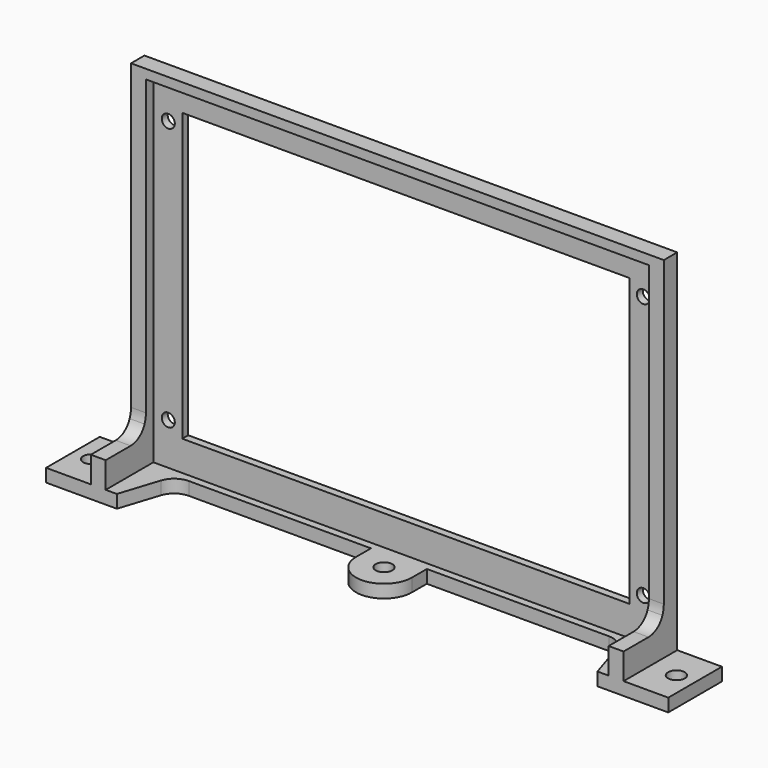
from build123d import *

# Parameters (mm, degrees)
F0_W      = 135
F0_H      = 90
F0_R      = 1.75
F0_W_2    = 120
F0_H_2    = 77
F1_DEPTH  = 2
F2_DEPTH  = 18
F3_R      = 2.25
F4_DEPTH  = 25
F5_DEPTH  = 1.5
F7_DEPTH  = 143.001
F8_W      = 12
F8_H      = 18
F9_DEPTH  = 3.5
F10_R     = 2.25
F11_DEPTH = 3.501
F12_R     = 2.25
F13_DEPTH = 3.501
F14_W     = 135
F14_H     = 2.5
F15_DEPTH = 2.5


# Not quite as in the source:
# - a feature names something its author has since deleted; it is built from what else it names


with BuildPart() as f1:
    # F0 (on Front) → F1 (new body)
    with BuildSketch(Plane.XZ):
        with Locations((41.872507602, -14.5468179137)):
            Rectangle(F0_W, F0_H)
        with Locations((-21.627492398, -49.7468179137)):
            Circle(F0_R, mode=Mode.SUBTRACT)
        with Locations((105.872507602, -49.7468179137)):
            Circle(F0_R, mode=Mode.SUBTRACT)
        with Locations((-21.627492398, 20.8531820863)):
            Circle(F0_R, mode=Mode.SUBTRACT)
        with Locations((42.122507602, -14.4468179137)):
            Rectangle(F0_W_2, F0_H_2, mode=Mode.SUBTRACT)
        with Locations((105.872507602, 20.8531820863)):
            Circle(F0_R, mode=Mode.SUBTRACT)
    extrude(amount=F1_DEPTH)

    # F0 (on Front) → F2 (join)
    with BuildSketch(Plane.XZ):
        Polygon((-25.627492398, -59.5468179137), (-25.627492398, 30.4531820863), (-29.627492398, 30.4531820863), (-29.627492398, -64.5468179137), (113.372507602, -64.5468179137), (113.372507602, 30.4531820863), (109.372507602, 30.4531820863), (109.372507602, -59.5468179137), align=None)
    extrude(amount=F2_DEPTH)

    # F3 (on face) → F4 (cut)
    with BuildSketch(Plane(origin=(0, 0, -64.5468179137), x_dir=(1, 0, 0), z_dir=(0, 0, -1))):
        with Locations((-9.627492398, 9)):
            Circle(F3_R)
        with Locations((41.872507602, 9)):
            Circle(F3_R)
        with Locations((93.372507602, 9)):
            Circle(F3_R)
    extrude(amount=-F4_DEPTH, mode=Mode.SUBTRACT)

    # F5 (cut): a face of the model
    f5_faces = [f1.faces().sort_by_distance(p)[0] for p in [
        (41.872507602, -3.3594484176, -59.5468179137),
    ]]
    extrude(f5_faces, amount=-F5_DEPTH, mode=Mode.SUBTRACT)

    # F6 (on face) → F7 (cut, through all)
    with BuildSketch(Plane.YZ.offset(113.372507602)):
        with BuildLine():
            Line((-18, 30.4531820863), (-18, -54.0468179137))
            Line((-18, -54.0468179137), (-9.6275595227, -54.0468179137))
            ThreePointArc((-9.6275595227, -54.0468179137), (-6.7891073566, -53.1630284647), (-4.9540928207, -50.8240936338))
            ThreePointArc((-4.9540928207, -50.8240936338), (-4.6144653792, -49.6089954864), (-4.5, -48.3525290189))
            Line((-4.5, -48.3525290189), (-4.5, 30.4531820863))
            Line((-4.5, 30.4531820863), (-18, 30.4531820863))
        make_face()
    extrude(amount=-F7_DEPTH, mode=Mode.SUBTRACT)

    # F8 (on face) → F9 (join, through all)
    with BuildSketch(Plane(origin=(0, 0, -64.5468179137), x_dir=(1, 0, 0), z_dir=(0, 0, -1))):
        with Locations((-35.627492398, 9)):
            Rectangle(F8_W, F8_H)
        with Locations((119.372507602, 9)):
            Rectangle(F8_W, F8_H)
    extrude(amount=-F9_DEPTH)

    # F10 (on face) → F11 (cut, through all)
    with BuildSketch(Plane.XY.offset(-61.0468179137)):
        with Locations((-36.627492398, -9)):
            Circle(F10_R)
        with Locations((120.372507602, -9)):
            Circle(F10_R)
    extrude(amount=-F11_DEPTH, mode=Mode.SUBTRACT)

    # F12 (on face) → F13 (cut, through all)
    with BuildSketch(Plane.XY.offset(-61.0468179137)):
        with BuildLine():
            Line((34.372507602, -4), (-14.4826919802, -4))
            ThreePointArc((-14.4826919802, -4), (-17.4280077943, -4.959565029), (-19.2428347866, -7.4699540979))
            Line((-19.2428347866, -7.4699540979), (-22.627492398, -18))
            Line((-22.627492398, -18), (106.372507602, -18))
            Line((106.372507602, -18), (102.9878499906, -7.4699540979))
            ThreePointArc((102.9878499906, -7.4699540979), (101.1730229983, -4.959565029), (98.2277071842, -4))
            Line((98.2277071842, -4), (49.372507602, -4))
            Line((49.372507602, -4), (49.372507602, -9))
            ThreePointArc((49.372507602, -9), (41.872507602, -16.5), (34.372507602, -9))
            Line((34.372507602, -9), (34.372507602, -4))
        make_face()
        with Locations((-9.627492398, -9)):
            Circle(F12_R, mode=Mode.SUBTRACT)
        with Locations((93.372507602, -9)):
            Circle(F12_R, mode=Mode.SUBTRACT)
    extrude(amount=-F13_DEPTH, mode=Mode.SUBTRACT)

    # F14 (on face) → F15 (join)
    with BuildSketch(Plane.XY.offset(30.4531820863)):
        with Locations((41.872507602, -3.25)):
            Rectangle(F14_W, F14_H)
        Polygon((-29.627492398, -4.5), (-25.627492398, -4.5), (-25.627492398, -2), (109.372507602, -2), (109.372507602, -4.5), (113.372507602, -4.5), (113.372507602, 0), (-29.627492398, 0), align=None)
    extrude(amount=F15_DEPTH)


solid = f1.part
